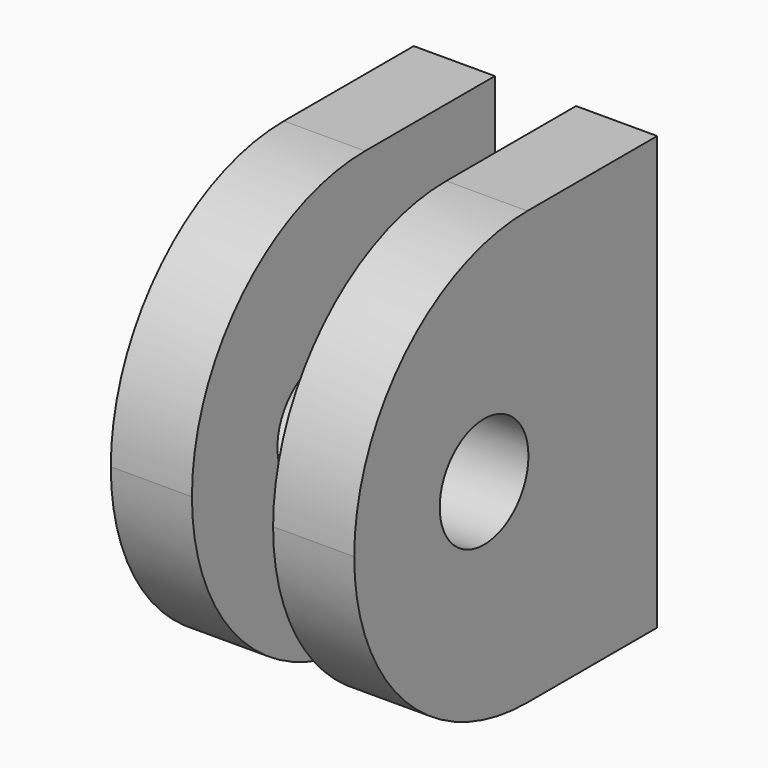
from build123d import *

# Parameters (mm, degrees)
F0_W     = 15
F0_H     = 80
F1_DEPTH = 70
F2_R     = 39.99999
F2_2_R   = 39.99999
F3_R     = 10.25
F4_DEPTH = 86.5
F5_R     = 10.25
F6_DEPTH = 25


# Not quite as in the source:
# - a fillet or chamfer is up to 0.001 mm smaller than in the source, because OpenCascade refuses the exact size


with BuildPart() as f1:
    # F0 (on Front) → F1 (new body)
    with BuildSketch(Plane.XZ):
        with Locations((5.25, 36)):
            Rectangle(F0_W, F0_H)
    extrude(amount=F1_DEPTH)

    # F2 (radius 40 in the source; OpenCascade refuses exactly that, so slightly less here)
    f2_edges = [f1.edges().sort_by_distance(p)[0] for p in [
        (5.25, -70, 76),
        (5.25, -70, -4),
    ]]
    fillet(f2_edges, radius=F2_R)


with BuildPart() as f1b:
    # F0 (on Front) → F1, piece 2 (new body)
    with BuildSketch(Plane.XZ):
        with Locations((35.25, 36)):
            Rectangle(F0_W, F0_H)
    extrude(amount=F1_DEPTH)

    # F2#2 (radius 40 in the source; OpenCascade refuses exactly that, so slightly less here)
    f2_2_edges = [f1b.edges().sort_by_distance(p)[0] for p in [
        (35.25, -70, 76),
        (35.25, -70, -4),
    ]]
    fillet(f2_2_edges, radius=F2_2_R)


with BuildPart() as f4_tool:
    # F3 (on face) → F4 (new body)
    with BuildSketch(Plane.YZ.offset(42.75)):
        with Locations((-40, 36)):
            Circle(F3_R)
    extrude(amount=-F4_DEPTH)


with BuildPart() as f1_1:
    add(f1.part)

    # F4: cut by f4_tool
    add(f4_tool.part, mode=Mode.SUBTRACT)

    # F5 (on face) → F6 (cut)
    with BuildSketch(Plane(origin=(-2.25, 0, 0), x_dir=(0, -1, 0), z_dir=(-1, 0, 0))):
        with Locations((40, 36)):
            Circle(F5_R)
    extrude(amount=-F6_DEPTH, mode=Mode.SUBTRACT)


with BuildPart() as f1b_1:
    add(f1b.part)

    # F4: cut by f4_tool
    add(f4_tool.part, mode=Mode.SUBTRACT)


solid = Compound([f1_1.part, f1b_1.part])
